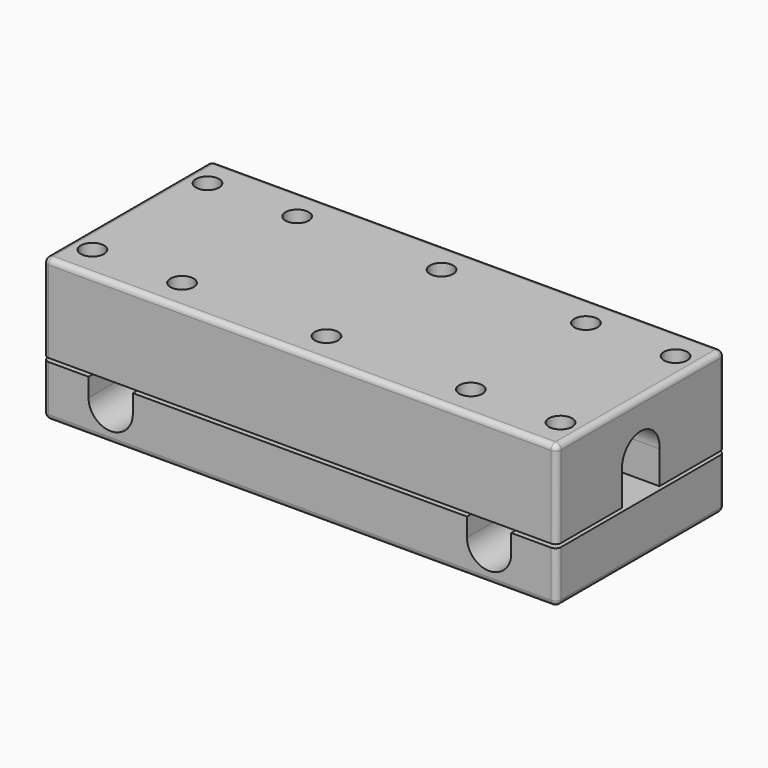
from build123d import *

# Parameters (mm, degrees)
F1_DEPTH  = 25.8
F4_DEPTH  = 92.801
F3_W      = 60.4
F3_H      = 0.65
F3_W_2    = 8.2
F5_DEPTH  = 38.001
F8_DEPTH  = 24.1
F11_DEPTH = 24.1
F12_R     = 1
F13_D     = 4.2


with BuildPart() as f1:
    # F0 (on Top) → F1 (new body)
    with BuildSketch(Plane.XY):
        Polygon((-94.1600755115, 24.7224580343), (-94.1600755115, -13.2775419657), (-85.9600755115, -13.2775419657), (-77.9600755115, -13.2775419657), (-47.7600755115, -13.2775419657), (-47.7600755115, 24.7224580343), align=None)
        Polygon((-1.3600755115, 24.7224580343), (-47.7600755115, 24.7224580343), (-47.7600755115, -13.2775419657), (-17.5600755115, -13.2775419657), (-9.5600755115, -13.2775419657), (-1.3600755115, -13.2775419657), align=None)
    extrude(amount=F1_DEPTH)

    # F2 (on face) → F4 (cut, through all)
    with BuildSketch(Plane(origin=(-94.1600755115, 0, 0), x_dir=(0, -1, 0), z_dir=(-1, 0, 0))):
        with BuildLine():
            ThreePointArc((-1.4724589241, 16.247249813), (-1.4724582568, 16.2486249064), (-1.4724580343, 16.25))
            ThreePointArc((-1.4724580343, 16.25), (-5.8677825168, 20.4975146609), (-9.9625195848, 15.9595210024))
            ThreePointArc((-9.9625195848, 15.9595210024), (-5.5785078489, 12.0024385415), (-1.4724589241, 16.247249813))
        make_face()
        with BuildLine():
            ThreePointArc((-1.4724589241, 16.247249813), (-5.5785078489, 12.0024385415), (-9.9625195848, 15.9595210024))
            Line((-9.9625195848, 15.9595210024), (-9.9625195848, 10.0030505006))
            ThreePointArc((-9.9625195848, 10.0030505006), (-9.3894148029, 9.6503084877), (-8.7871766185, 9.35))
            Line((-8.7871766185, 9.35), (-2.6577394502, 9.35))
            ThreePointArc((-2.6577394502, 9.35), (-2.0502502399, 9.6532288266), (-1.4724589241, 10.0098070892))
            Line((-1.4724589241, 10.0098070892), (-1.4724589241, 16.247249813))
        make_face()
        with BuildLine():
            ThreePointArc((-8.7871766185, 9.35), (-9.3894148029, 9.6503084877), (-9.9625195848, 10.0030505006))
            Line((-9.9625195848, 10.0030505006), (-9.9625195848, 9.35))
            Line((-9.9625195848, 9.35), (-8.7871766185, 9.35))
        make_face()
        with BuildLine():
            Line((-1.4724589241, 9.35), (-1.4724589241, 10.0098070892))
            ThreePointArc((-1.4724589241, 10.0098070892), (-2.0502502399, 9.6532288266), (-2.6577394502, 9.35))
            Line((-2.6577394502, 9.35), (-1.4724589241, 9.35))
        make_face()
    extrude(amount=-F4_DEPTH, mode=Mode.SUBTRACT)

    # F3 (on face) → F5 (cut, through all)
    with BuildSketch(Plane.XZ.offset(13.2775419657)):
        with BuildLine():
            ThreePointArc((-84.145824811, 9.35), (-85.4773896287, 7.9048625675), (-85.9600755115, 6))
            Line((-85.9600755115, 6), (-77.9600755115, 6))
            ThreePointArc((-77.9600755115, 6), (-78.4427613944, 7.9048625675), (-79.7743262121, 9.35))
            Line((-79.7743262121, 9.35), (-84.145824811, 9.35))
        make_face()
        with BuildLine():
            ThreePointArc((-81.9600755115, 10), (-83.1002509366, 9.8340579025), (-84.145824811, 9.35))
            Line((-84.145824811, 9.35), (-79.7743262121, 9.35))
            ThreePointArc((-79.7743262121, 9.35), (-80.8199000864, 9.8340579025), (-81.9600755115, 10))
        make_face()
        with BuildLine():
            Line((-11.3743262121, 9.35), (-15.745824811, 9.35))
            ThreePointArc((-15.745824811, 9.35), (-17.0773896287, 7.9048625675), (-17.5600755115, 6))
            Line((-17.5600755115, 6), (-9.5600755115, 6))
            ThreePointArc((-9.5600755115, 6), (-10.0427613944, 7.9048625675), (-11.3743262121, 9.35))
        make_face()
        with BuildLine():
            ThreePointArc((-13.560075504, 10), (-14.700250933, 9.8340579036), (-15.745824811, 9.35))
            Line((-15.745824811, 9.35), (-11.3743262121, 9.35))
            ThreePointArc((-11.3743262121, 9.35), (-12.4199000828, 9.8340579015), (-13.560075504, 10))
        make_face()
        with BuildLine():
            Line((-77.9600755115, 6), (-85.9600755115, 6))
            ThreePointArc((-85.9600755115, 6), (-81.9600755115, 2), (-77.9600755115, 6))
        make_face()
        with BuildLine():
            ThreePointArc((-79.7743262121, 9.35), (-78.4427613944, 7.9048625675), (-77.9600755115, 6))
            Line((-77.9600755115, 6), (-77.9600755115, 9.35))
            Line((-77.9600755115, 9.35), (-79.7743262121, 9.35))
        make_face()
        with BuildLine():
            ThreePointArc((-81.9600755115, 10), (-80.8199000864, 9.8340579025), (-79.7743262121, 9.35))
            Line((-79.7743262121, 9.35), (-77.9600755115, 9.35))
            Line((-77.9600755115, 9.35), (-77.9600755115, 10))
            Line((-77.9600755115, 10), (-81.9600755115, 10))
        make_face()
        with BuildLine():
            Line((-85.9600755115, 9.35), (-84.145824811, 9.35))
            ThreePointArc((-84.145824811, 9.35), (-83.1002509366, 9.8340579025), (-81.9600755115, 10))
            Line((-81.9600755115, 10), (-85.9600755115, 10))
            Line((-85.9600755115, 10), (-85.9600755115, 9.35))
        make_face()
        with BuildLine():
            Line((-85.9600755115, 9.35), (-85.9600755115, 6))
            ThreePointArc((-85.9600755115, 6), (-85.4773896287, 7.9048625675), (-84.145824811, 9.35))
            Line((-84.145824811, 9.35), (-85.9600755115, 9.35))
        make_face()
        with BuildLine():
            Line((-9.5600755115, 6), (-17.5600755115, 6))
            ThreePointArc((-17.5600755115, 6), (-13.5600755115, 2), (-9.5600755115, 6))
        make_face()
        with BuildLine():
            Line((-17.5600755115, 10), (-17.5600755115, 9.35))
            Line((-17.5600755115, 9.35), (-15.745824811, 9.35))
            ThreePointArc((-15.745824811, 9.35), (-14.700250933, 9.8340579036), (-13.560075504, 10))
            Line((-13.560075504, 10), (-17.5600755115, 10))
        make_face()
        with BuildLine():
            Line((-15.745824811, 9.35), (-17.5600755115, 9.35))
            Line((-17.5600755115, 9.35), (-17.5600755115, 6))
            ThreePointArc((-17.5600755115, 6), (-17.0773896287, 7.9048625675), (-15.745824811, 9.35))
        make_face()
        with BuildLine():
            Line((-9.5600755115, 9.35), (-11.3743262121, 9.35))
            ThreePointArc((-11.3743262121, 9.35), (-10.0427613944, 7.9048625675), (-9.5600755115, 6))
            Line((-9.5600755115, 6), (-9.5600755115, 9.35))
        make_face()
        with BuildLine():
            Line((-9.5600755115, 10), (-13.560075504, 10))
            ThreePointArc((-13.560075504, 10), (-12.4199000828, 9.8340579015), (-11.3743262121, 9.35))
            Line((-11.3743262121, 9.35), (-9.5600755115, 9.35))
            Line((-9.5600755115, 9.35), (-9.5600755115, 10))
        make_face()
        with Locations((-47.7600755115, 9.675)):
            Rectangle(F3_W, F3_H)
        with Locations((-90.0600755115, 9.675)):
            Rectangle(F3_W_2, F3_H)
        with Locations((-5.4600755115, 9.675)):
            Rectangle(F3_W_2, F3_H)
    extrude(amount=-F5_DEPTH, mode=Mode.SUBTRACT)

    # F7 (on line) → F8 (cut)
    with BuildSketch(Plane(origin=(-75.9600755115, 0, 0), x_dir=(0, -1, 0), z_dir=(-1, 0, 0))):
        with BuildLine():
            ThreePointArc((-8.7871766185, 9.35), (-12.0525893643, 12.1351564617), (-13.2724580343, 16.25))
            Line((-13.2724580343, 16.25), (-13.2724580343, 9.35))
            Line((-13.2724580343, 9.35), (-8.7871766185, 9.35))
        make_face()
        with BuildLine():
            Line((1.8275419657, 9.35), (1.8275419657, 16.25))
            ThreePointArc((1.8275419657, 16.25), (0.6076732957, 12.1351564617), (-2.6577394502, 9.35))
            Line((-2.6577394502, 9.35), (1.8275419657, 9.35))
        make_face()
        with BuildLine():
            ThreePointArc((-2.6577394502, 9.35), (0.6076732957, 12.1351564617), (1.8275419657, 16.25))
            Line((1.8275419657, 16.25), (-13.2724580343, 16.25))
            ThreePointArc((-13.2724580343, 16.25), (-12.0525893643, 12.1351564617), (-8.7871766185, 9.35))
            Line((-8.7871766185, 9.35), (-2.6577394502, 9.35))
        make_face()
        with BuildLine():
            Line((-13.2724580343, 16.25), (1.8275419657, 16.25))
            ThreePointArc((1.8275419657, 16.25), (-5.7224580343, 23.8), (-13.2724580343, 16.25))
        make_face()
        with BuildLine():
            ThreePointArc((-8.7871766185, 9.35), (-5.7224580343, 8.7), (-2.6577394502, 9.35))
            Line((-2.6577394502, 9.35), (-8.7871766185, 9.35))
        make_face()
    extrude(amount=-F8_DEPTH, mode=Mode.SUBTRACT)

    # F10 (on line) → F11 (cut)
    with BuildSketch(Plane(origin=(-19.5600755115, 0, 0), x_dir=(0, -1, 0), z_dir=(-1, 0, 0))):
        with BuildLine():
            Line((-13.2724580343, 16.25), (1.8275419657, 16.25))
            ThreePointArc((1.8275419657, 16.25), (-5.7224580343, 23.8), (-13.2724580343, 16.25))
        make_face()
        with BuildLine():
            ThreePointArc((-2.6577394502, 9.35), (0.6076732957, 12.1351564617), (1.8275419657, 16.25))
            Line((1.8275419657, 16.25), (-13.2724580343, 16.25))
            ThreePointArc((-13.2724580343, 16.25), (-12.0525893643, 12.1351564617), (-8.7871766185, 9.35))
            Line((-8.7871766185, 9.35), (-2.6577394502, 9.35))
        make_face()
        with BuildLine():
            ThreePointArc((-8.7871766185, 9.35), (-12.0525893643, 12.1351564617), (-13.2724580343, 16.25))
            Line((-13.2724580343, 16.25), (-13.2724580343, 9.35))
            Line((-13.2724580343, 9.35), (-8.7871766185, 9.35))
        make_face()
        with BuildLine():
            Line((1.8275419657, 9.35), (1.8275419657, 16.25))
            ThreePointArc((1.8275419657, 16.25), (0.6076732957, 12.1351564617), (-2.6577394502, 9.35))
            Line((-2.6577394502, 9.35), (1.8275419657, 9.35))
        make_face()
        with BuildLine():
            ThreePointArc((-8.7871766185, 9.35), (-5.7224580343, 8.7), (-2.6577394502, 9.35))
            Line((-2.6577394502, 9.35), (-8.7871766185, 9.35))
        make_face()
    extrude(amount=F11_DEPTH, mode=Mode.SUBTRACT)

    # F12
    f12_edges = [f1.edges().sort_by_distance(p)[0] for p in [
        (-47.760076, -13.277542, 0),
        (-1.360076, 5.722458, 0),
        (-94.160076, 5.722458, 0),
        (-47.760076, 24.722458, 25.8),
        (-47.760076, -13.277542, 25.8),
        (-1.360076, 5.722458, 25.8),
        (-1.360076, 24.722458, 17.9),
        (-1.360076, -13.277542, 17.9),
        (-94.160076, 5.722458, 25.8),
        (-94.160076, -13.277542, 17.9),
        (-94.160076, 24.722458, 17.9),
        (-47.760076, 24.722458, 0),
        (-94.160076, 24.722458, 4.675),
        (-94.160076, -13.277542, 4.675),
        (-1.360076, 24.722458, 4.675),
        (-1.360076, -13.277542, 4.675),
    ]]
    fillet(f12_edges, radius=F12_R)

    # F13 (through all)
    with Locations(Plane(origin=(0, 0, 0), x_dir=(1, 0, 0), z_dir=(0, 0, -1))):
        with Locations((-47.7600755115, -18.7224580343), (-47.7600755115, 7.2775419657), (-90.0600755115, 7.2775419657), (-5.4600755115, 7.2775419657), (-5.4600755115, -18.7224580343), (-21.6600755115, -18.7224580343), (-73.8600755115, -18.7224580343), (-90.0600755115, -18.7224580343), (-73.8600755115, 7.2775419657), (-21.6600755115, 7.2775419657)):
            Hole(F13_D / 2)


solid = f1.part
